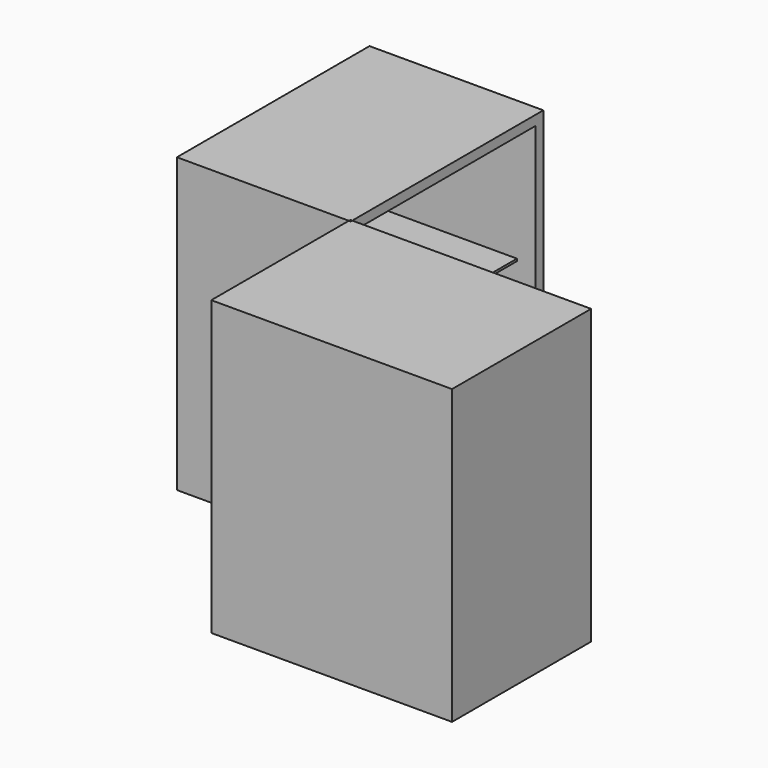
from build123d import *

# Parameters (mm, degrees)
F1_DEPTH = 76.2
F2_T     = -2.54
F3_T     = -2.54
F4_W     = 57.5280706716
F4_H     = 0.5833022296
F5_DEPTH = 37.846


# Not quite as in the source:
# - the program builds the solid bodies; features that only make, move or delete a surface that nothing else refers to are left out


with BuildPart() as f1:
    # F0 (on Top) → F1 (new body)
    with BuildSketch(Plane.XY):
        Polygon((0, -0.486087054), (0, 0), (0.4860870778, 0), (0.4860901141, 62.1219835938), (-44.7200468874, 62.1219858033), (-44.7200499475, -0.4860848683), align=None)
    extrude(amount=F1_DEPTH)

    # F2
    f2_openings = [f1.faces().sort_by_distance(p)[0] for p in [
        (0.486089, 31.060992, 38.1),
    ]]
    offset(amount=F2_T, openings=f2_openings, kind=Kind.INTERSECTION)

    # F4 (on face) → F5 (join)
    with BuildSketch(Plane(origin=(-42.1800499237, 2.0616e-06, 0), x_dir=(4.89e-08, 1, 0), z_dir=(1, -4.89e-08, 0))):
        with Locations((30.8179482818, 41.4146538824)):
            Rectangle(F4_W, F4_H)
    extrude(amount=F5_DEPTH)


with BuildPart() as f1b:
    # F0 (on Top) → F1, piece 2 (new body)
    with BuildSketch(Plane.XY):
        Polygon((62.6080706716, 0), (0.4860870778, 0), (0.486087054, -0.4860870778), (0, -0.486087054), (0, -45.2061370015), (62.6080706716, -45.2061370015), align=None)
    extrude(amount=F1_DEPTH)

    # F3
    f3_openings = [f1b.faces().sort_by_distance(p)[0] for p in [
        (31.547079, 0, 38.1),
    ]]
    offset(amount=F3_T, openings=f3_openings, kind=Kind.INTERSECTION)


solid = Compound([f1.part, f1b.part])
